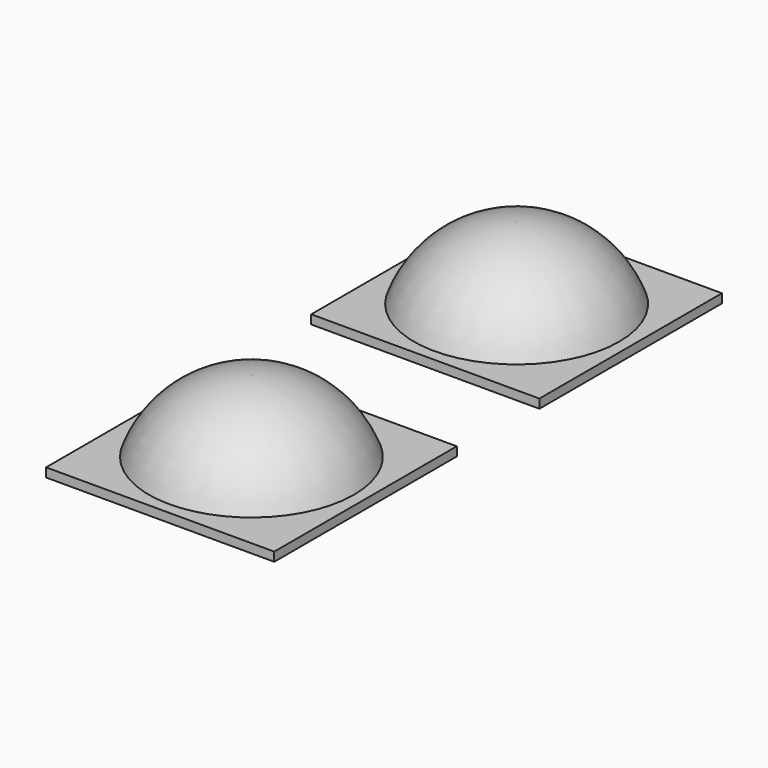
from build123d import *

# Parameters (mm, degrees)
F0_W     = 25.4
F0_H     = 25.4
F0_R     = 11.43
F1_DEPTH = 1
F0_R_2   = 10.16
F2_DEPTH = 9


# Not quite as in the source:
# - a fillet or chamfer that OpenCascade refuses, or shapes differently, is made with other operations: its cross-section is extruded or revolved along the edge and cut away or added


with BuildPart() as f1:
    # F0 (on Top) → F1 (new body)
    with BuildSketch(Plane.XY):
        Rectangle(F0_W, F0_H)
        Circle(F0_R, mode=Mode.SUBTRACT)
    extrude(amount=F1_DEPTH)

    # F0 (on Top) → F2 (join)
    with BuildSketch(Plane.XY):
        Circle(F0_R)
        Circle(F0_R_2, mode=Mode.SUBTRACT)
        Circle(F0_R_2)
    extrude(amount=F2_DEPTH)

    # F3: fillet of radius 12.1 on 1 edges, made by hand

    # F3_s1 → F3_t2 (revolve, cut)
    with BuildSketch(Plane.XZ):
        with BuildLine():
            ThreePointArc((11.43, 1), (7.0028112758, 6.8), (0.0458004234, 9))
            Line((0.0458004234, 9), (0.0458004234, 9.242))
            Line((0.0458004234, 9.242), (11.43, 9.242))
            Line((11.43, 9.242), (11.672, 9))
            ThreePointArc((11.672, 9), (11.672, 5), (11.6576839915, 1.082))
            Line((11.6576839915, 1.082), (11.43, 1))
        make_face()
    revolve(axis=Axis((0, 0, 9), (0, 0, 1)), mode=Mode.SUBTRACT)


with BuildPart() as f4_1:
    # F4: copy of F1
    add(f1.part.moved(Location((0, 36.89959, 0))))


solid = Compound([f1.part, f4_1.part])
